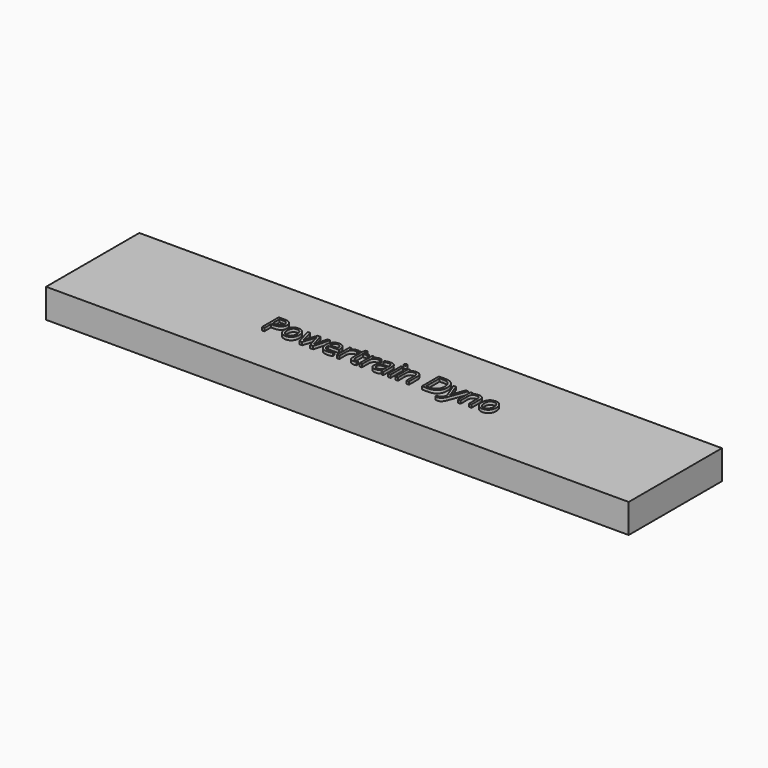
from build123d import *

# Parameters (mm, degrees)
F1_DEPTH     = 250
F2_TEXT_SIZE = 254.5642575872
F3_DEPTH     = 25.4


# Not quite as in the source:
# - Text() gives the source's letters only with a copy of the font that has no kerning and outlines rounded to 1/6400 em; it was checked with that copy


with BuildPart() as f1:
    # F0 (on Top) → F1 (new body)
    with BuildSketch(Plane.XY):
        Polygon((-2500, -500), (2500, -500), (2500, 500), (500, 500), (-500, 500), (-2500, 500), align=None)
    extrude(amount=F1_DEPTH)

    # F2 (on face) → F3 (join)
    with BuildSketch(Plane.XY.offset(250)):
        with Locations((-1000, -91.8184797016)):
            Text('Powertrain Dyno', F2_TEXT_SIZE, font='Open Sans', text_align=(TextAlign.LEFT, TextAlign.BOTTOM))
    extrude(amount=F3_DEPTH)


solid = f1.part
